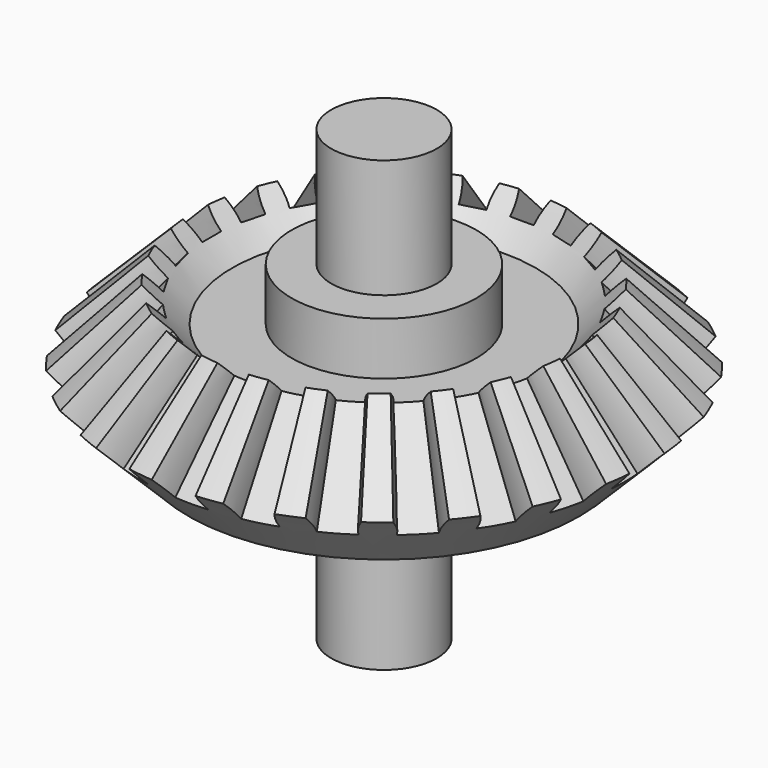
from build123d import *

# Parameters (mm, degrees)
F6_COPIES_COUNT = 24


# Not quite as in the source:
# - a pattern or mirror of a feature is missing from the dataset's text; its kind, count and spacing are read off the source's solid


with BuildPart() as f2:
    # F1 (on Front) → F2 (revolve)
    with BuildSketch(Plane.XZ):
        Polygon((0, 8), (0, 0), (14.8284271247, 0), (20, 5.1715728753), (14.3431457505, 10.8284271247), (11.5147186258, 8), align=None)
    revolve(axis=Axis((0, 0, 0), (0, 0, -1)))

    # F4 (on line) → F6 section 0
    with BuildSketch(Plane(origin=(7.4142135624, 0, -7.4142135624), x_dir=(0.7071067812, 0, 0.7071067812), z_dir=(0.7071067812, 0, -0.7071067812)), mode=Mode.PRIVATE) as f6_s0:
        with BuildLine():
            ThreePointArc((20.2989898732, 3.1598300563), (17.9751555465, 1.7437073078), (15.2989898732, 1.25))
            Line((15.2989898732, 1.25), (15.2989898732, -1.25))
            ThreePointArc((15.2989898732, -1.25), (17.9751555465, -1.7437073078), (20.2989898732, -3.1598300563))
            Line((20.2989898732, -3.1598300563), (20.2989898732, 3.1598300563))
        make_face()
    f6 = loft([f6_s0.sketch, Vertex(0, 0, 25.1715728753)], mode=Mode.SUBTRACT)

    # F6_copies: F6 ×24 about axis
    f6_copies_axis = Axis((0, 0, 0), (0, 0, 1))
    for i in range(1, F6_COPIES_COUNT):
        add(f6.rotate(f6_copies_axis, i * 360 / F6_COPIES_COUNT), mode=Mode.SUBTRACT)

    # F7 (on Front) → F8 (revolve)
    with BuildSketch(Plane.XZ):
        Polygon((7, 12), (4, 12), (4, 21), (0, 21), (0, -13), (4, -13), (4, -2), (7, -2), align=None)
    revolve(axis=Axis((0, 0, 0), (0, 0, -1)))


solid = f2.part
